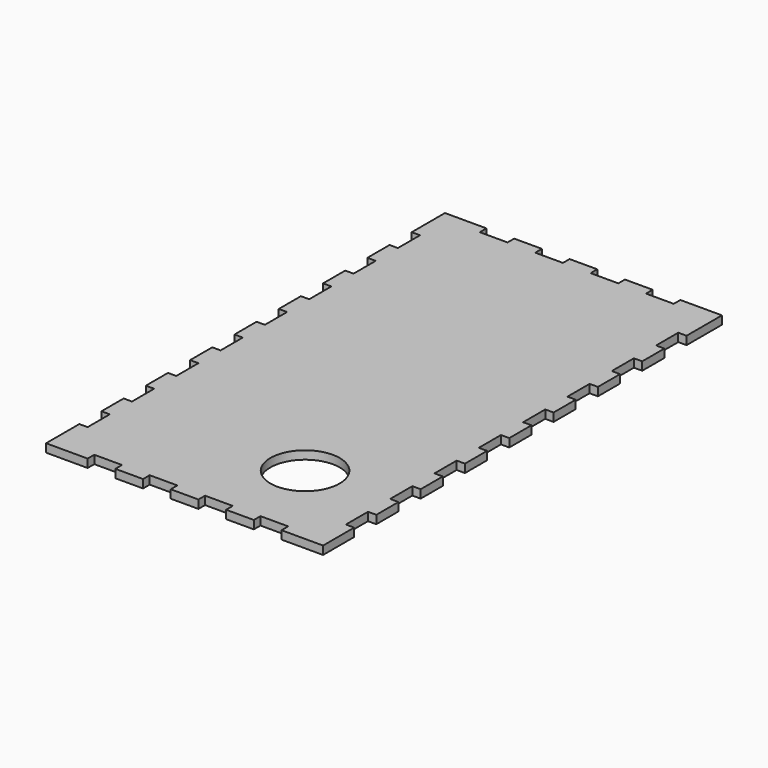
from build123d import *

# Parameters (mm, degrees)
F0_R     = 12.5
F1_DEPTH = 1.5


# Not quite as in the source:
# - ends of sketch curves that miss each other by under 0.0002 mm in the source are joined


with BuildPart() as f1:
    # F0 (on Top) → F1 (new body, symmetric)
    with BuildSketch(Plane.XY):
        Polygon((-46.9999983907, 3.8743e-06), (-46.9999983907, -4.9999961257), (-43.9999983907, -4.9999961257), (-43.9999983907, -14.9999961257), (-46.9999983907, -14.9999961257), (-46.9999983907, -24.9999961257), (-43.9999983907, -24.9999961257), (-43.9999983907, -34.9999961257), (-46.9999983907, -34.9999961257), (-46.9999983907, -44.9999961257), (-43.9999983907, -44.9999961257), (-43.9999983907, -54.9999961257), (-46.9999983907, -54.9999961257), (-46.9999983907, -64.9999961257), (-43.9999983907, -64.9999961257), (-43.9999983907, -74.9999961257), (-46.9999983907, -74.9999961257), (-46.9999983907, -89.9999961257), (-31.9999983907, -89.9999961257), (-31.9999983907, -86.9999961257), (-21.9999983907, -86.9999961257), (-21.9999983907, -89.9999961257), (-11.9999983907, -89.9999961257), (-11.9999983907, -86.9999961257), (-1.9999983907, -86.9999961257), (-1.9999983907, -89.9999961257), (8.0000016093, -89.9999961257), (8.0000016093, -86.9999961257), (18.0000016093, -86.9999961257), (18.0000016093, -89.9999961257), (28.0000016093, -89.9999961257), (28.0000016093, -86.9999961257), (38.0000016093, -86.9999961257), (38.0000016093, -89.9999961257), (53.0000016093, -89.9999961257), (53.0000030994, -75.968132019), (50.0000030994, -75.968132019), (50.0000030994, -65.968132019), (53.0000030994, -65.968132019), (53.0000030994, -55.968132019), (50.0000030994, -55.968132019), (50.0000030994, -45.968132019), (53.0000030994, -45.968132019), (53.0000030994, -35.968132019), (50.0000030994, -35.968132019), (50.0000030994, -25.968132019), (53.0000030994, -25.968132019), (53.0000030994, -15.968132019), (50.0000030994, -15.968132019), (50.0000030994, -5.968132019), (53.0000030994, -5.968132019), (53.0000030994, 3.8743e-06), (53.0000030994, 4.031867981), (50.0000030994, 4.031867981), (50.0000030994, 14.031867981), (53.0000030994, 14.031867981), (53.0000030994, 24.031867981), (50.0000030994, 24.031867981), (50.0000030994, 34.031867981), (53.0000030994, 34.031867981), (53.0000030994, 44.031867981), (50.0000030994, 44.031867981), (50.0000030994, 54.031867981), (53.0000030994, 54.031867981), (53.0000030994, 64.031867981), (50.0000030994, 64.031867981), (50.0000030994, 74.031867981), (53.0000030994, 74.031867981), (53.0000030994, 90.0000038743), (38.0000016093, 90.0000035763), (38.0000016093, 87.0000035763), (28.0000016093, 87.0000035763), (28.0000016093, 90.0000035763), (18.0000016093, 90.0000035763), (18.0000016093, 87.0000035763), (8.0000016093, 87.0000035763), (8.0000016093, 90.0000035763), (-1.9999983907, 90.0000035763), (-1.9999983907, 87.0000035763), (-11.9999983907, 87.0000035763), (-11.9999983907, 90.0000035763), (-21.9999983907, 90.0000035763), (-21.9999983907, 87.0000035763), (-31.9999983907, 87.0000035763), (-31.9999983907, 90.0000035763), (-46.9999983907, 90.0000035763), (-46.9999983907, 75.0000038743), (-43.9999983907, 75.0000038743), (-43.9999983907, 65.0000038743), (-46.9999983907, 65.0000038743), (-46.9999983907, 55.0000038743), (-43.9999983907, 55.0000038743), (-43.9999983907, 45.0000038743), (-46.9999983907, 45.0000038743), (-46.9999983907, 35.0000038743), (-43.9999983907, 35.0000038743), (-43.9999983907, 25.0000038743), (-46.9999983907, 25.0000038743), (-46.9999983907, 15.0000038743), (-43.9999983907, 15.0000038743), (-43.9999983907, 5.0000038743), (-46.9999983907, 5.0000038743), align=None)
        with Locations((20.5000030994, -57.4999969183)):
            Circle(F0_R, mode=Mode.SUBTRACT)
    extrude(amount=F1_DEPTH, both=True)


solid = f1.part
